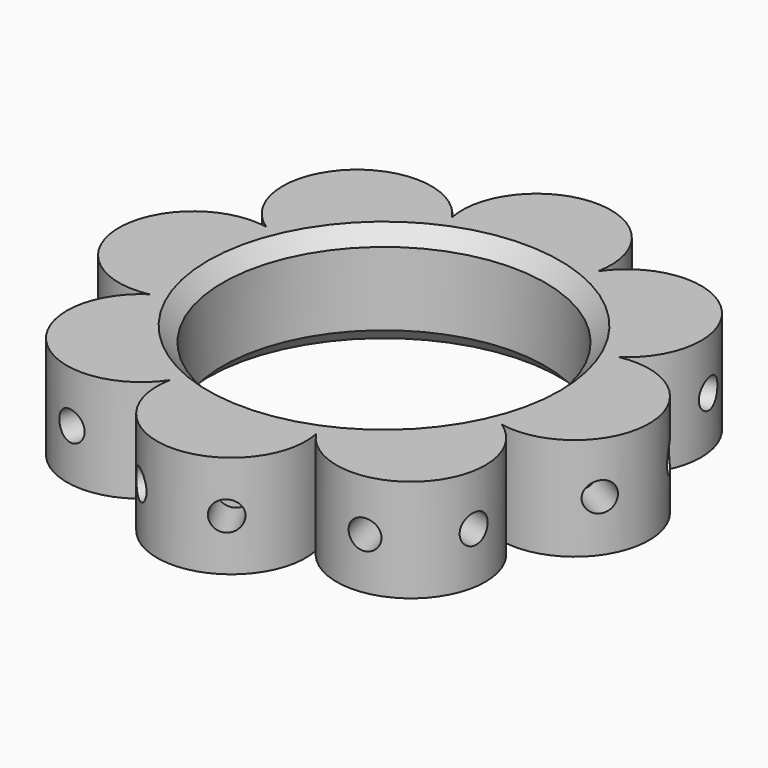
from build123d import *

# Parameters (mm, degrees)
F0_R             = 11
F1_DEPTH         = 3.5
F2_SIZE          = 1
F6_R             = 1
F7_DEPTH         = 7
F7_COPIES_COUNT  = 8
F9_R             = 1
F10_DEPTH        = 7
F10_COPIES_COUNT = 8


# Not quite as in the source:
# - a pattern or mirror of a feature is missing from the dataset's text; its kind, count and spacing are read off the source's solid


with BuildPart() as f1:
    # F0 (on Top) → F1 (new body, symmetric)
    with BuildSketch(Plane.XY):
        with BuildLine():
            ThreePointArc((12.0104759307, 4.9747832032), (12.750219353, 2.5361203541), (13, 0))
            ThreePointArc((13, 0), (12.750219353, -2.5361203541), (12.0104759307, -4.9747832032))
            ThreePointArc((12.0104759307, -4.9747832032), (12.0107097924, -4.9749394725), (12.0109436454, -4.9750957548))
            ThreePointArc((12.0109436454, -4.9750957548), (18.0724560365, 0), (12.0109436454, 4.9750957548))
            ThreePointArc((12.0109436454, 4.9750957548), (12.0107097924, 4.9749394725), (12.0104759307, 4.9747832032))
        make_face()
        with BuildLine():
            ThreePointArc((12.0103919138, 4.974986038), (12.0104339226, 4.9748846207), (12.0104759307, 4.9747832032))
            ThreePointArc((12.0104759307, 4.9747832032), (12.0107097924, 4.9749394725), (12.0109436454, 4.9750957548))
            ThreePointArc((12.0109436454, 4.9750957548), (12.0106677781, 4.975040904), (12.0103919138, 4.974986038))
        make_face()
        with BuildLine():
            ThreePointArc((12.0109436454, -4.9750957548), (12.0107097924, -4.9749394725), (12.0104759307, -4.9747832032))
            ThreePointArc((12.0104759307, -4.9747832032), (12.0104339226, -4.9748846207), (12.0103919138, -4.974986038))
            ThreePointArc((12.0103919138, -4.974986038), (12.0106677781, -4.975040904), (12.0109436454, -4.9750957548))
        make_face()
        with BuildLine():
            ThreePointArc((4.974986038, 12.0103919138), (9.1923881554, 9.1923881554), (12.0103919138, 4.974986038))
            ThreePointArc((12.0103919138, 4.974986038), (12.0106677781, 4.975040904), (12.0109436454, 4.9750957548))
            ThreePointArc((12.0109436454, 4.9750957548), (12.7791562161, 12.7791562161), (4.9750957548, 12.0109436454))
            ThreePointArc((4.9750957548, 12.0109436454), (4.975040904, 12.0106677781), (4.974986038, 12.0103919138))
        make_face()
        with BuildLine():
            ThreePointArc((12.0109436454, -4.9750957548), (12.0106677781, -4.975040904), (12.0103919138, -4.974986038))
            ThreePointArc((12.0103919138, -4.974986038), (9.1923881554, -9.1923881554), (4.974986038, -12.0103919138))
            ThreePointArc((4.974986038, -12.0103919138), (4.975040904, -12.0106677781), (4.9750957548, -12.0109436454))
            ThreePointArc((4.9750957548, -12.0109436454), (12.7791562161, -12.7791562161), (12.0109436454, -4.9750957548))
        make_face()
        with BuildLine():
            ThreePointArc((4.9747832032, 12.0104759307), (4.9748846207, 12.0104339226), (4.974986038, 12.0103919138))
            ThreePointArc((4.974986038, 12.0103919138), (4.975040904, 12.0106677781), (4.9750957548, 12.0109436454))
            ThreePointArc((4.9750957548, 12.0109436454), (4.9749394725, 12.0107097924), (4.9747832032, 12.0104759307))
        make_face()
        with BuildLine():
            ThreePointArc((4.9747832032, 12.0104759307), (4.9749394725, 12.0107097924), (4.9750957548, 12.0109436454))
            ThreePointArc((4.9750957548, 12.0109436454), (0, 18.0724560365), (-4.9750957548, 12.0109436454))
            ThreePointArc((-4.9750957548, 12.0109436454), (-4.9749394725, 12.0107097924), (-4.9747832032, 12.0104759307))
            ThreePointArc((-4.9747832032, 12.0104759307), (0, 13), (4.9747832032, 12.0104759307))
        make_face()
        with BuildLine():
            ThreePointArc((4.9750957548, -12.0109436454), (4.975040904, -12.0106677781), (4.974986038, -12.0103919138))
            ThreePointArc((4.974986038, -12.0103919138), (4.9748846207, -12.0104339226), (4.9747832032, -12.0104759307))
            ThreePointArc((4.9747832032, -12.0104759307), (4.9749394725, -12.0107097924), (4.9750957548, -12.0109436454))
        make_face()
        with BuildLine():
            ThreePointArc((-4.9750957548, -12.0109436454), (0, -18.0724560365), (4.9750957548, -12.0109436454))
            ThreePointArc((4.9750957548, -12.0109436454), (4.9749394725, -12.0107097924), (4.9747832032, -12.0104759307))
            ThreePointArc((4.9747832032, -12.0104759307), (0, -13), (-4.9747832032, -12.0104759307))
            ThreePointArc((-4.9747832032, -12.0104759307), (-4.9749394725, -12.0107097924), (-4.9750957548, -12.0109436454))
        make_face()
        with BuildLine():
            ThreePointArc((-4.9747832032, 12.0104759307), (-4.9749394725, 12.0107097924), (-4.9750957548, 12.0109436454))
            ThreePointArc((-4.9750957548, 12.0109436454), (-4.975040904, 12.0106677781), (-4.974986038, 12.0103919138))
            ThreePointArc((-4.974986038, 12.0103919138), (-4.9748846207, 12.0104339226), (-4.9747832032, 12.0104759307))
        make_face()
        with BuildLine():
            ThreePointArc((-4.974986038, 12.0103919138), (-4.975040904, 12.0106677781), (-4.9750957548, 12.0109436454))
            ThreePointArc((-4.9750957548, 12.0109436454), (-12.7791562161, 12.7791562161), (-12.0109436454, 4.9750957548))
            ThreePointArc((-12.0109436454, 4.9750957548), (-12.0106677781, 4.975040904), (-12.0103919138, 4.974986038))
            ThreePointArc((-12.0103919138, 4.974986038), (-9.1923881554, 9.1923881554), (-4.974986038, 12.0103919138))
        make_face()
        with BuildLine():
            ThreePointArc((-4.974986038, -12.0103919138), (-4.975040904, -12.0106677781), (-4.9750957548, -12.0109436454))
            ThreePointArc((-4.9750957548, -12.0109436454), (-4.9749394725, -12.0107097924), (-4.9747832032, -12.0104759307))
            ThreePointArc((-4.9747832032, -12.0104759307), (-4.9748846207, -12.0104339226), (-4.974986038, -12.0103919138))
        make_face()
        with BuildLine():
            ThreePointArc((-12.0109436454, -4.9750957548), (-12.7791562161, -12.7791562161), (-4.9750957548, -12.0109436454))
            ThreePointArc((-4.9750957548, -12.0109436454), (-4.975040904, -12.0106677781), (-4.974986038, -12.0103919138))
            ThreePointArc((-4.974986038, -12.0103919138), (-9.1923881554, -9.1923881554), (-12.0103919138, -4.974986038))
            ThreePointArc((-12.0103919138, -4.974986038), (-12.0106677781, -4.975040904), (-12.0109436454, -4.9750957548))
        make_face()
        with BuildLine():
            ThreePointArc((-12.0103919138, 4.974986038), (-12.0106677781, 4.975040904), (-12.0109436454, 4.9750957548))
            ThreePointArc((-12.0109436454, 4.9750957548), (-12.0107097924, 4.9749394725), (-12.0104759307, 4.9747832032))
            ThreePointArc((-12.0104759307, 4.9747832032), (-12.0104339226, 4.9748846207), (-12.0103919138, 4.974986038))
        make_face()
        with BuildLine():
            ThreePointArc((-12.0104759307, 4.9747832032), (-12.0107097924, 4.9749394725), (-12.0109436454, 4.9750957548))
            ThreePointArc((-12.0109436454, 4.9750957548), (-18.0724560365, 0), (-12.0109436454, -4.9750957548))
            ThreePointArc((-12.0109436454, -4.9750957548), (-12.0107097924, -4.9749394725), (-12.0104759307, -4.9747832032))
            ThreePointArc((-12.0104759307, -4.9747832032), (-13, 0), (-12.0104759307, 4.9747832032))
        make_face()
        with BuildLine():
            ThreePointArc((-12.0104759307, -4.9747832032), (-12.0107097924, -4.9749394725), (-12.0109436454, -4.9750957548))
            ThreePointArc((-12.0109436454, -4.9750957548), (-12.0106677781, -4.975040904), (-12.0103919138, -4.974986038))
            ThreePointArc((-12.0103919138, -4.974986038), (-12.0104339226, -4.9748846207), (-12.0104759307, -4.9747832032))
        make_face()
        with BuildLine():
            ThreePointArc((12.0104759307, -4.9747832032), (12.750219353, -2.5361203541), (13, 0))
            ThreePointArc((13, 0), (12.750219353, 2.5361203541), (12.0104759307, 4.9747832032))
            ThreePointArc((12.0104759307, 4.9747832032), (12.0104339226, 4.9748846207), (12.0103919138, 4.974986038))
            ThreePointArc((12.0103919138, 4.974986038), (9.1923881554, 9.1923881554), (4.974986038, 12.0103919138))
            ThreePointArc((4.974986038, 12.0103919138), (4.9748846207, 12.0104339226), (4.9747832032, 12.0104759307))
            ThreePointArc((4.9747832032, 12.0104759307), (0, 13), (-4.9747832032, 12.0104759307))
            ThreePointArc((-4.9747832032, 12.0104759307), (-4.9748846207, 12.0104339226), (-4.974986038, 12.0103919138))
            ThreePointArc((-4.974986038, 12.0103919138), (-9.1923881554, 9.1923881554), (-12.0103919138, 4.974986038))
            ThreePointArc((-12.0103919138, 4.974986038), (-12.0104339226, 4.9748846207), (-12.0104759307, 4.9747832032))
            ThreePointArc((-12.0104759307, 4.9747832032), (-13, 0), (-12.0104759307, -4.9747832032))
            ThreePointArc((-12.0104759307, -4.9747832032), (-12.0104339226, -4.9748846207), (-12.0103919138, -4.974986038))
            ThreePointArc((-12.0103919138, -4.974986038), (-9.1923881554, -9.1923881554), (-4.974986038, -12.0103919138))
            ThreePointArc((-4.974986038, -12.0103919138), (-4.9748846207, -12.0104339226), (-4.9747832032, -12.0104759307))
            ThreePointArc((-4.9747832032, -12.0104759307), (0, -13), (4.9747832032, -12.0104759307))
            ThreePointArc((4.9747832032, -12.0104759307), (4.9748846207, -12.0104339226), (4.974986038, -12.0103919138))
            ThreePointArc((4.974986038, -12.0103919138), (9.1923881554, -9.1923881554), (12.0103919138, -4.974986038))
            ThreePointArc((12.0103919138, -4.974986038), (12.0104339226, -4.9748846207), (12.0104759307, -4.9747832032))
        make_face()
        Circle(F0_R, mode=Mode.SUBTRACT)
    extrude(amount=F1_DEPTH, both=True)

    # F2
    f2_edges = [f1.edges().sort_by_distance(p)[0] for p in [
        (-11, 0, 3.5),
        (-11, 0, -3.5),
    ]]
    chamfer(f2_edges, length=F2_SIZE)

    # F6 (on line) → F7 (cut)
    with BuildSketch(Plane(origin=(-5.2779168675, 19.6974539077, 0), x_dir=(-0.9659258263, -0.2588190451, 0), z_dir=(-0.2588190451, 0.9659258263, 0))):
        with Locations((6, 0)):
            Circle(F6_R)
    f7 = extrude(amount=-F7_DEPTH, mode=Mode.SUBTRACT)

    # F7_copies: F7 ×8 about axis
    f7_copies_axis = Axis((0, 0, 0), (0, 0, 1))
    for i in range(1, F7_COPIES_COUNT):
        add(f7.rotate(f7_copies_axis, i * 360 / F7_COPIES_COUNT), mode=Mode.SUBTRACT)

    # F9 (on line) → F10 (cut)
    with BuildSketch(Plane(origin=(-19.6974539077, 5.2779168675, 0), x_dir=(-0.2588190451, -0.9659258263, 0), z_dir=(-0.9659258263, 0.2588190451, 0))):
        with Locations((-6, 0)):
            Circle(F9_R)
    f10 = extrude(amount=-F10_DEPTH, mode=Mode.SUBTRACT)

    # F10_copies: F10 ×8 about axis
    f10_copies_axis = Axis((0, 0, 0), (0, 0, 1))
    for i in range(1, F10_COPIES_COUNT):
        add(f10.rotate(f10_copies_axis, i * 360 / F10_COPIES_COUNT), mode=Mode.SUBTRACT)


solid = f1.part
